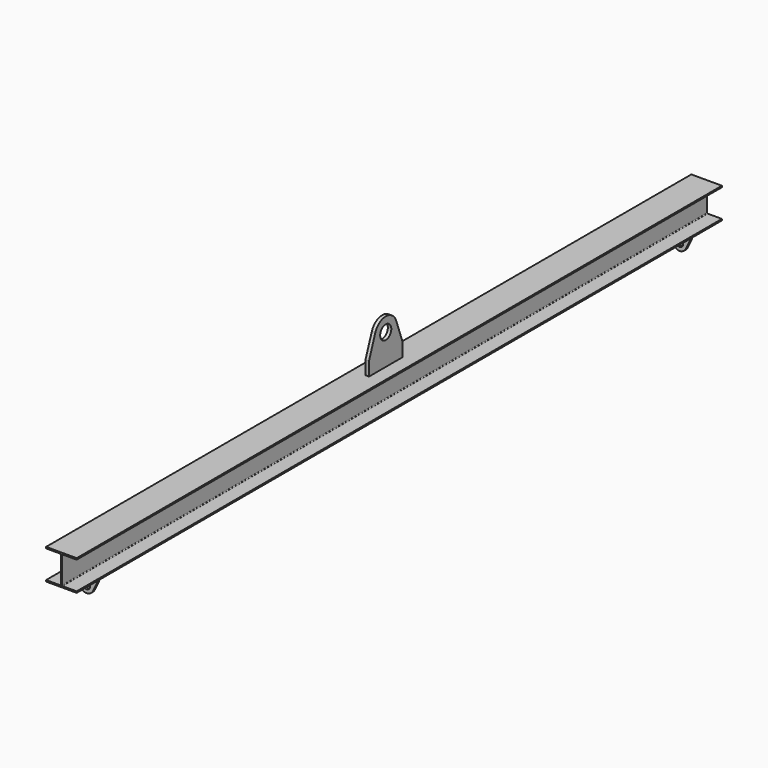
from build123d import *

# Parameters (mm, degrees)
F1_DEPTH = 2900
F2_R     = 50
F3_DEPTH = 12.5
F5_R     = 25
F6_DEPTH = 8


# Not quite as in the source:
# - a pattern or mirror of a feature is missing from the dataset's text; its kind, count and spacing are read off the source's solid


with BuildPart() as f1:
    # F0 (on Front) → F1 (new body, symmetric)
    with BuildSketch(Plane.XZ):
        with BuildLine():
            Line((110, 110), (0, 110))
            Line((0, 110), (-110, 110))
            Line((-110, 110), (-110, 100))
            Line((-110, 100), (-9, 100))
            ThreePointArc((-9, 100), (-5.4644660941, 98.5355339059), (-4, 95))
            Line((-4, 95), (-4, 0))
            Line((-4, 0), (-4, -95))
            ThreePointArc((-4, -95), (-5.4644660941, -98.5355339059), (-9, -100))
            Line((-9, -100), (-110, -100))
            Line((-110, -100), (-110, -110))
            Line((-110, -110), (0, -110))
            Line((0, -110), (110, -110))
            Line((110, -110), (110, -100))
            Line((110, -100), (9, -100))
            ThreePointArc((9, -100), (5.4644660941, -98.5355339059), (4, -95))
            Line((4, -95), (4, 0))
            Line((4, 0), (4, 95))
            ThreePointArc((4, 95), (5.4644660941, 98.5355339059), (9, 100))
            Line((9, 100), (110, 100))
            Line((110, 100), (110, 110))
        make_face()
    extrude(amount=F1_DEPTH, both=True)

    # F2 (on Right) → F3 (join, symmetric)
    with BuildSketch(Plane.YZ):
        with BuildLine():
            Line((-150, 210), (-150, 110))
            Line((-150, 110), (150, 110))
            Line((150, 110), (150, 210))
            Line((150, 210), (93.9877055833, 364.1512986458))
            ThreePointArc((93.9877055833, 364.1512986458), (0, 430), (-93.9877055833, 364.1512986458))
            Line((-93.9877055833, 364.1512986458), (-150, 210))
        make_face()
        with Locations((0, 330)):
            Circle(F2_R, mode=Mode.SUBTRACT)
    extrude(amount=F3_DEPTH, both=True)

    # F5 (on offset) → F6 (join, symmetric)
    with BuildSketch(Plane.XZ.offset(2665)):
        with BuildLine():
            Line((75, -110), (-75, -110))
            Line((-75, -110), (-75, -150))
            Line((-75, -150), (-44.9795530586, -211.836661985))
            ThreePointArc((-44.9795530586, -211.836661985), (0, -240), (44.9795530586, -211.836661985))
            Line((44.9795530586, -211.836661985), (75, -150))
            Line((75, -150), (75, -110))
        make_face()
        with Locations((0, -190)):
            Circle(F5_R, mode=Mode.SUBTRACT)
    f6 = extrude(amount=F6_DEPTH, both=True)

    # F6_copies: F6 across plane
    add(f6.mirror(Plane.ZX))


solid = f1.part
